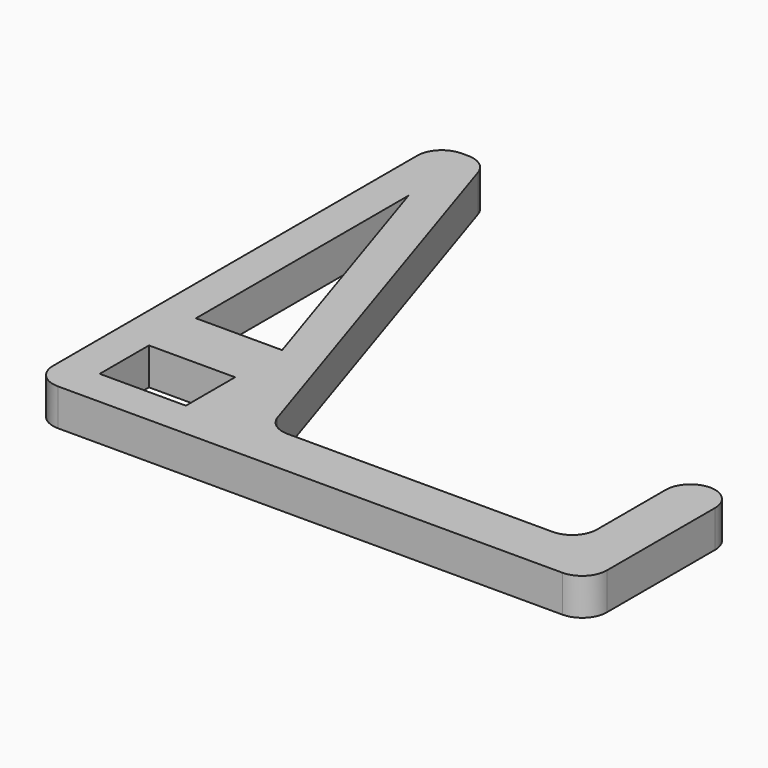
from build123d import *

# Parameters (mm, degrees)
F0_W     = 7
F0_H     = 5
F1_DEPTH = 3
F2_R     = 1.99999


# Not quite as in the source:
# - a fillet or chamfer is up to 0.001 mm smaller than in the source, because OpenCascade refuses the exact size
# - a feature names something its author has since deleted; it is built from what else it names


with BuildPart() as f1:
    # F0 (on Top) → F1 (new body)
    with BuildSketch(Plane.XY):
        Polygon((25, 0), (0, 0), (-12, 37), (-16, 37), (-16, -4), (29, -4), (29, 11), (25, 11), align=None)
        with Locations((-9.5, 1.5)):
            Rectangle(F0_W, F0_H, mode=Mode.SUBTRACT)
        Polygon((-13, 8.7756748306), (-13, 30.3590081639), (-6, 8.7756748306), align=None, mode=Mode.SUBTRACT)
    extrude(amount=F1_DEPTH)

    # F2 (radius 2 in the source; OpenCascade refuses exactly that, so slightly less here)
    f2_edges = [f1.edges().sort_by_distance(p)[0] for p in [
        (-16, -4, 1.5),
        (25, 0, 1.5),
        (-12, 37, 1.5),
        (29, 11, 1.5),
        (0, 0, 1.5),
        (-16, 37, 1.5),
        (29, -4, 1.5),
        (25, 11, 1.5),
    ]]
    fillet(f2_edges, radius=F2_R)


solid = f1.part
